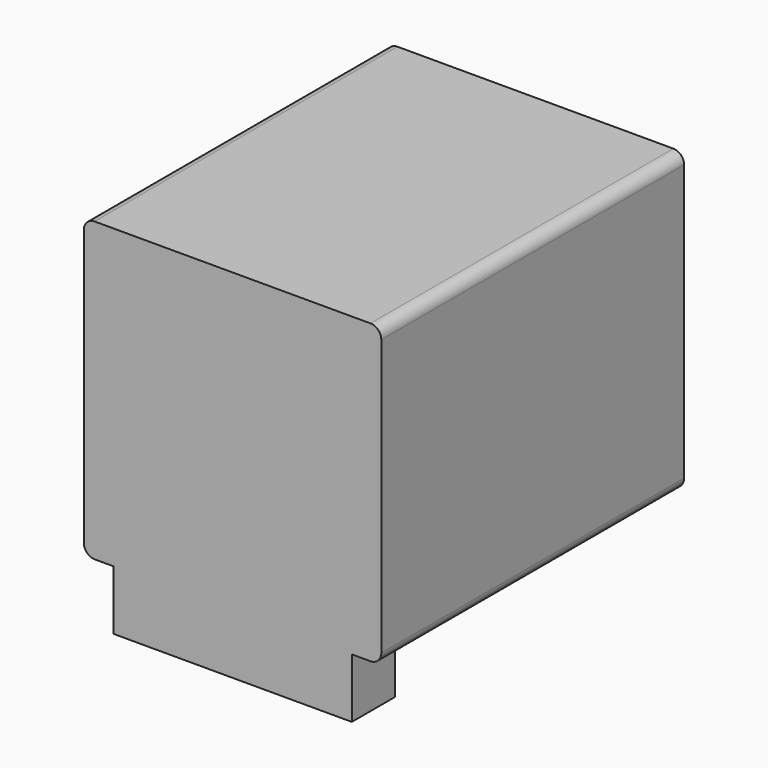
from build123d import *

# Parameters (mm, degrees)
F1_DEPTH    = 4
F2_R        = 2
F0_W        = 10
F0_H        = 10
F3_DEPTH    = 11
F4_W        = 44.1
F4_H        = 10
F5_DEPTH    = 55
F6_T        = 1.5
F6_T3_DEPTH = 13
F6_T5_DEPTH = 47.1
F6_T7_DEPTH = 7
F6_T9_DEPTH = 27.1
F7_R        = 2


# Not quite as in the source:
# - a shell that OpenCascade refuses in one call is made with other operations: the cavity is built on its own and cut out


with BuildPart() as f1:
    # F0 (on Top) → F1 (new body)
    with BuildSketch(Plane.XY):
        Polygon((-12.05, 0), (0, 0), (12.05, 0), (12.05, 10), (-12.05, 10), align=None)
        Polygon((-12.05, 48.5), (-12.05, 10), (12.05, 10), (12.05, 48.5), (8.55, 45), (10.55, 45), (10.55, 23), (0, 23), (-10.55, 23), (-10.55, 45), (-8.55, 45), align=None)
    extrude(amount=F1_DEPTH)

    # F2
    f2_edges = [f1.edges().sort_by_distance(p)[0] for p in [
        (-10.55, 23, 2),
        (10.55, 23, 2),
    ]]
    fillet(f2_edges, radius=F2_R)

    # F0 (on Top) → F3 (join)
    with BuildSketch(Plane.XY):
        with Locations((17.05, 5)):
            Rectangle(F0_W, F0_H)
        Polygon((-12.05, 0), (0, 0), (12.05, 0), (12.05, 10), (-12.05, 10), align=None)
        with Locations((-17.05, 5)):
            Rectangle(F0_W, F0_H)
    extrude(amount=F3_DEPTH)

    # F4 (on face) → F5 (join)
    with BuildSketch(Plane.XY.offset(11)):
        Polygon((-27.5, 70), (-27.5, 0), (-22.05, 0), (-22.05, 10), (22.05, 10), (22.05, 0), (27.5, 0), (27.5, 70), align=None)
        with Locations((0, 5)):
            Rectangle(F4_W, F4_H)
    extrude(amount=F5_DEPTH)

    # F6: shell of thickness 1.5, made by hand


with BuildPart() as f6_core1:
    # F6_t2: copy of F1
    add(f1.part)

    # the walls: a layer under each face that stays
    f6_faces = [f6_core1.faces().sort_by_distance(p)[0] for p in [
        (-27.5, 35, 38.5),
        (0, 0, 33),
        (0, 35, 11),
        (0, 35, 66),
        (27.5, 35, 38.5),
        (22.05, 5, 5.5),
        (0, 10, 5.5),
        (-22.05, 5, 5.5),
        (-14.7, 8.0833333333, 0),
        (12.05, 29.25, 2),
        (-8.0333333333, 16.4166666667, 4),
        (-12.05, 29.25, 2),
        (10.55, 35, 2),
        (9.9642135624, 23.5857864376, 2),
        (0, 23, 2),
        (-9.9642135624, 23.5857864376, 2),
        (-10.55, 35, 2),
        (-9.55, 45, 2),
        (-10.3, 46.75, 2),
        (10.3, 46.75, 2),
        (9.55, 45, 2),
    ]]
    thicken(f6_faces, amount=-F6_T, mode=Mode.SUBTRACT)

    # F6_s4 → F6_t3 (cut)
    with BuildSketch(Plane.XZ.offset(-11.5)):
        Polygon((22.065, 10.985), (22.05, 12.5), (20.55, 12.5), (20.55, 11), align=None)
        Polygon((-22.065, 10.985), (-22.05, 12.5), (-20.55, 12.5), (-20.55, 11), align=None)
    extrude(amount=F6_T3_DEPTH, mode=Mode.SUBTRACT)

    # F6_s6 → F6_t5 (cut)
    with BuildSketch(Plane.YZ.offset(-23.55)):
        Polygon((10.015, 10.985), (10, 12.5), (8.5, 12.5), (8.5, 11), align=None)
    extrude(amount=F6_T5_DEPTH, mode=Mode.SUBTRACT)

    # F6_s8 → F6_t7 (cut)
    with BuildSketch(Plane.XY.offset(-1.5)):
        Polygon((12.065, 10.015), (12.05, 8.5), (10.55, 8.5), (10.55, 10), align=None)
        Polygon((-12.065, 10.015), (-12.05, 8.5), (-10.55, 8.5), (-10.55, 10), align=None)
        Polygon((10.535, 44.985), (12.05, 45), (12.05, 46.5), (10.55, 46.5), align=None)
        Polygon((-10.535, 44.985), (-12.05, 45), (-12.05, 46.5), (-10.55, 46.5), align=None)
    extrude(amount=F6_T7_DEPTH, mode=Mode.SUBTRACT)

    # F6_s10 → F6_t9 (cut)
    with BuildSketch(Plane.YZ.offset(-13.55)):
        Polygon((10.015, 4.015), (8.5, 4), (8.5, 2.5), (10, 2.5), align=None)
    extrude(amount=F6_T9_DEPTH, mode=Mode.SUBTRACT)


with BuildPart() as f1_1:
    add(f1.part)

    # what is left inside the walls is the cavity
    f6_cavity = [f6_core1.part.solids().sort_by_distance(p)[0] for p in [
        (-25.985, 35.75, 47.166667),
    ]]
    add(f6_cavity, mode=Mode.SUBTRACT)

    # F7
    f7_edges = [f1_1.edges().sort_by_distance(p)[0] for p in [
        (-27.5, 35, 66),
        (-27.5, 35, 11),
        (27.5, 35, 11),
        (27.5, 35, 66),
    ]]
    fillet(f7_edges, radius=F7_R)


solid = f1_1.part
